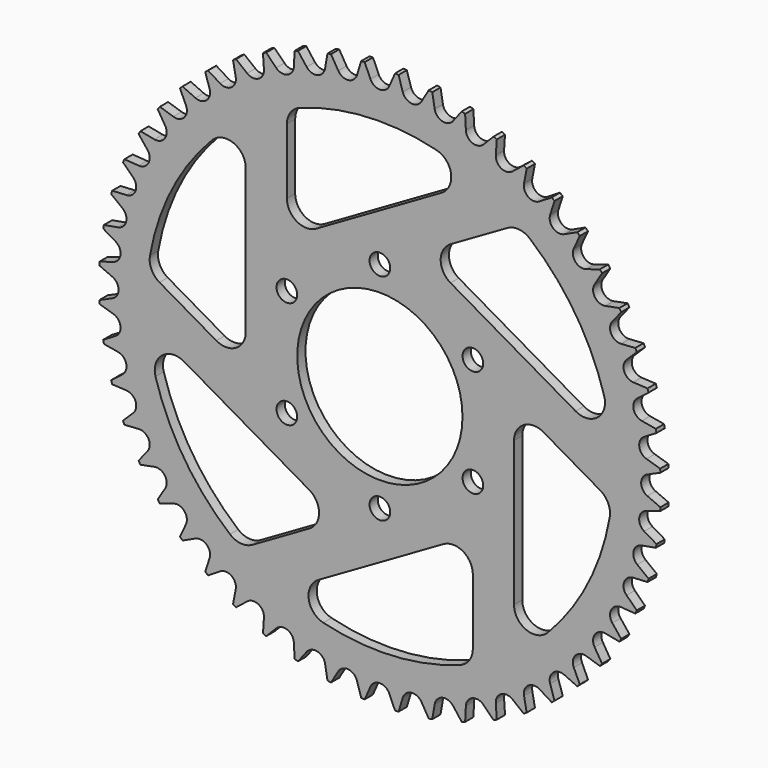
from build123d import *

# Parameters (mm, degrees)
F0_R            = 40
F0_R_2          = 5
F1_DEPTH        = 2.5
F2_DEPTH        = 12.5
F2_COPIES_COUNT = 6
F3_DEPTH        = 12.5
F3_COPIES_COUNT = 6
F4_DEPTH        = 12.5
F4_COPIES_COUNT = 52


# Not quite as in the source:
# - a pattern or mirror of a feature is missing from the dataset's text; its kind, count and spacing are read off the source's solid


with BuildPart() as f1:
    # F0 (on Front) → F1 (new body, symmetric)
    with BuildSketch(Plane.XZ):
        with BuildLine():
            Line((4.5765573956, -129.4862665507), (7.3550920645, -135.8009669359))
            ThreePointArc((7.3550920645, -135.8009669359), (0, 136), (-7.3550920645, -135.8009669359))
            Line((-7.3550920645, -135.8009669359), (-4.5765573956, -129.4862665507))
            ThreePointArc((-4.5765573956, -129.4862665507), (0, -126.5), (4.5765573956, -129.4862665507))
        make_face()
        with BuildLine():
            ThreePointArc((-30.75, 57.227241336), (-40.25, 57.227241336), (-45, 65.4544826719))
            Line((-45, 65.4544826719), (-45, 97.2213968219))
            ThreePointArc((-45, 97.2213968219), (-43.2847708383, 102.6663341948), (-38.7584541063, 106.1450999118))
            ThreePointArc((-38.7584541063, 106.1450999118), (-5.9596298031, 112.8427348685), (27.362218029, 109.6371699039))
            ThreePointArc((27.362218029, 109.6371699039), (34.4695521589, 101.740955732), (29.8118545664, 92.1926443725))
            Line((29.8118545664, 92.1926443725), (-30.75, 57.227241336))
        make_face(mode=Mode.SUBTRACT)
        Circle(F0_R, mode=Mode.SUBTRACT)
        with Locations((0, 52)):
            Circle(F0_R_2, mode=Mode.SUBTRACT)
        with BuildLine():
            Line((-45, 97.2213968219), (-45, 65.4544826719))
            ThreePointArc((-45, 65.4544826719), (-40.25, 57.227241336), (-30.75, 57.227241336))
            Line((-30.75, 57.227241336), (29.8118545664, 92.1926443725))
            ThreePointArc((29.8118545664, 92.1926443725), (34.4695521589, 101.740955732), (27.362218029, 109.6371699039))
            ThreePointArc((27.362218029, 109.6371699039), (-5.9596298031, 112.8427348685), (-38.7584541063, 106.1450999118))
            ThreePointArc((-38.7584541063, 106.1450999118), (-43.2847708383, 102.6663341948), (-45, 97.2213968219))
        make_face()
        with BuildLine():
            Line((7.4426687087, -136), (7.3550920645, -135.8009669359))
            Line((7.3550920645, -135.8009669359), (4.5765573956, -129.4862665507))
            ThreePointArc((4.5765573956, -129.4862665507), (0, -126.5), (-4.5765573956, -129.4862665507))
            Line((-4.5765573956, -129.4862665507), (-7.3550920645, -135.8009669359))
            Line((-7.3550920645, -135.8009669359), (-7.4426687087, -136))
            Line((-7.4426687087, -136), (7.4426687087, -136))
        make_face()
        with Locations((0, 52)):
            Circle(F0_R_2)
    extrude(amount=F1_DEPTH, both=True)

    # F0 (on Front) → F2 (cut, symmetric)
    with BuildSketch(Plane.XZ):
        with BuildLine():
            Line((-45, 97.2213968219), (-45, 65.4544826719))
            ThreePointArc((-45, 65.4544826719), (-40.25, 57.227241336), (-30.75, 57.227241336))
            Line((-30.75, 57.227241336), (29.8118545664, 92.1926443725))
            ThreePointArc((29.8118545664, 92.1926443725), (34.4695521589, 101.740955732), (27.362218029, 109.6371699039))
            ThreePointArc((27.362218029, 109.6371699039), (-5.9596298031, 112.8427348685), (-38.7584541063, 106.1450999118))
            ThreePointArc((-38.7584541063, 106.1450999118), (-43.2847708383, 102.6663341948), (-45, 97.2213968219))
        make_face()
    f2 = extrude(amount=F2_DEPTH, both=True, mode=Mode.SUBTRACT)

    # F2_copies: F2 ×6 about axis
    f2_copies_axis = Axis((0, 0, 0), (0, 1, 0))
    for i in range(1, F2_COPIES_COUNT):
        add(f2.rotate(f2_copies_axis, i * 360 / F2_COPIES_COUNT), mode=Mode.SUBTRACT)

    # F0 (on Front) → F3 (cut, symmetric)
    with BuildSketch(Plane.XZ):
        with Locations((0, 52)):
            Circle(F0_R_2)
    f3 = extrude(amount=F3_DEPTH, both=True, mode=Mode.SUBTRACT)

    # F3_copies: F3 ×6 about axis
    f3_copies_axis = Axis((0, 0, 0), (0, 1, 0))
    for i in range(1, F3_COPIES_COUNT):
        add(f3.rotate(f3_copies_axis, i * 360 / F3_COPIES_COUNT), mode=Mode.SUBTRACT)

    # F0 (on Front) → F4 (cut, symmetric)
    with BuildSketch(Plane.XZ):
        with BuildLine():
            Line((7.4426687087, -136), (7.3550920645, -135.8009669359))
            Line((7.3550920645, -135.8009669359), (4.5765573956, -129.4862665507))
            ThreePointArc((4.5765573956, -129.4862665507), (0, -126.5), (-4.5765573956, -129.4862665507))
            Line((-4.5765573956, -129.4862665507), (-7.3550920645, -135.8009669359))
            Line((-7.3550920645, -135.8009669359), (-7.4426687087, -136))
            Line((-7.4426687087, -136), (7.4426687087, -136))
        make_face()
    f4 = extrude(amount=F4_DEPTH, both=True, mode=Mode.SUBTRACT)

    # F4_copies: F4 ×52 about axis
    f4_copies_axis = Axis((0, 0, 0), (0, 1, 0))
    for i in range(1, F4_COPIES_COUNT):
        add(f4.rotate(f4_copies_axis, i * 360 / F4_COPIES_COUNT), mode=Mode.SUBTRACT)


solid = f1.part
